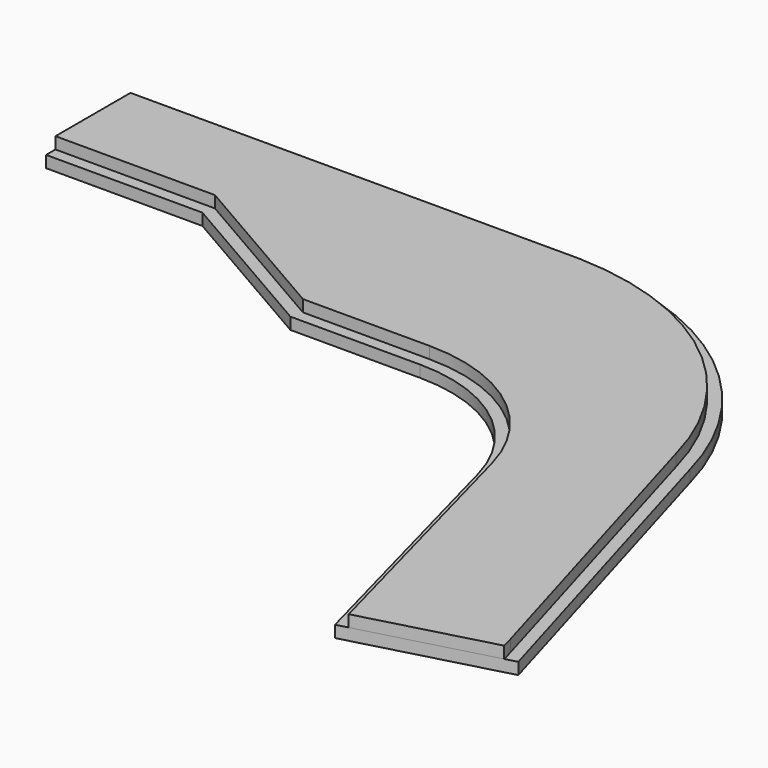
from build123d import *

# Parameters (mm, degrees)
F1_DEPTH = 3
F3_DEPTH = 3
F4_W     = 24
F4_H     = 3
F5_DEPTH = 3
F6_W     = 33.9326828589
F6_H     = 3
F7_DEPTH = 3


with BuildPart() as f1:
    # F0 (on Top) → F1 (new body)
    with BuildSketch(Plane.XY):
        with BuildLine():
            ThreePointArc((70.5214165197, -55.9710955009), (44.5935670538, -16.2265064733), (0, 0))
            Line((0, 0), (-115, 0))
            Line((-115, 0), (-115, -30))
            Line((-115, -30), (-75, -30))
            Line((-75, -30), (-33.1492031744, -54.1625688131))
            Line((-33.1492031744, -54.1625688131), (0, -54.1625688131))
            ThreePointArc((0, -54.1625688131), (24.3504571603, -62.4284352014), (38.6370330516, -83.809807009))
            Line((38.6370330516, -83.809807009), (57.1011837292, -152.7189554564))
            Line((57.1011837292, -152.7189554564), (95.7382167807, -142.3661936523))
            Line((95.7382167807, -142.3661936523), (70.5214165197, -55.9710955009))
        make_face()
    extrude(amount=-F1_DEPTH)

    # F2 (on face) → F3 (join)
    with BuildSketch(Plane.XY):
        with BuildLine():
            ThreePointArc((0, -51.1625688131), (26.1767414474, -60.0483751805), (41.5348105304, -83.0333498737))
            Line((41.5348105304, -83.0333498737), (59.2225040727, -149.0447208423))
            Line((59.2225040727, -149.0447208423), (91.9989588014, -140.262296267))
            Line((91.9989588014, -140.262296267), (67.629756974, -56.7711490177))
            ThreePointArc((67.629756974, -56.7711490177), (42.7604972061, -18.6017091288), (-0.0410552786, -3))
            Line((-0.0410552786, -3), (-112, -3))
            Line((-112, -3), (-112, -27))
            Line((-112, -27), (-74.1961524227, -27))
            Line((-74.1961524227, -27), (-32.3453555971, -51.1625688131))
            Line((-32.3453555971, -51.1625688131), (0, -51.1625688131))
        make_face()
    extrude(amount=F3_DEPTH)

    # F4 (on face) → F5 (join)
    with BuildSketch(Plane(origin=(-112, 0, 0), x_dir=(0, -1, 0), z_dir=(-1, 0, 0))):
        with Locations((15, 1.5)):
            Rectangle(F4_W, F4_H)
    extrude(amount=F5_DEPTH)

    # F6 (on face) → F7 (join)
    with BuildSketch(Plane(origin=(41.2283357456, -153.866243714, 0), x_dir=(0.9659258263, 0.2588190451, 0), z_dir=(0.2588190451, -0.9659258263, 0))):
        with Locations((35.5952752848, 1.5)):
            Rectangle(F6_W, F6_H)
    extrude(amount=F7_DEPTH)


solid = f1.part
